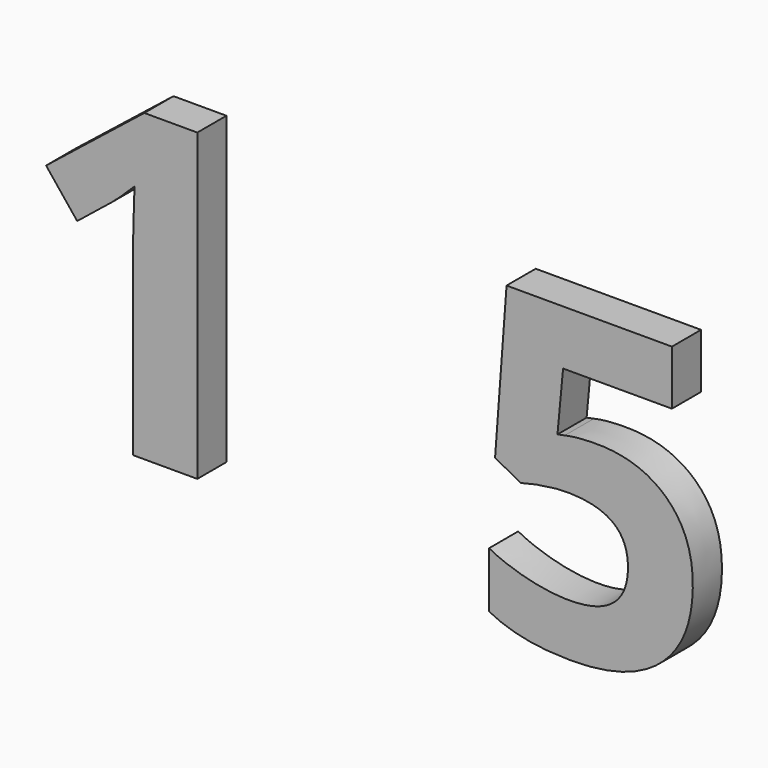
from build123d import *

# Parameters (mm, degrees)
F0_TEXT_SIZE = 74.4517038889
F1_DEPTH     = 6.35
F2_TEXT_SIZE = 74.4517038889
F3_DEPTH     = 6.35


# Not quite as in the source:
# - Text() gives the source's letters only with a copy of the font that has no kerning and outlines rounded to 1/6400 em; it was checked with that copy


with BuildPart() as f1:
    # F0 (on Front) → F1 (new body)
    with BuildSketch(Plane.XZ):
        with Locations((-100.2669684631, -16.2812282581)):
            Text('1', F0_TEXT_SIZE, font='Open Sans', font_style=FontStyle.BOLD, text_align=(TextAlign.LEFT, TextAlign.BOTTOM))
    extrude(amount=F1_DEPTH)


with BuildPart() as f3:
    # F2 (on Front) → F3 (new body)
    with BuildSketch(Plane.XZ):
        with Locations((-22.2900758798, -22.2278998835)):
            Text('5', F2_TEXT_SIZE, font='Open Sans', font_style=FontStyle.BOLD, text_align=(TextAlign.LEFT, TextAlign.BOTTOM))
    extrude(amount=F3_DEPTH)


solid = Compound([f1.part, f3.part])
